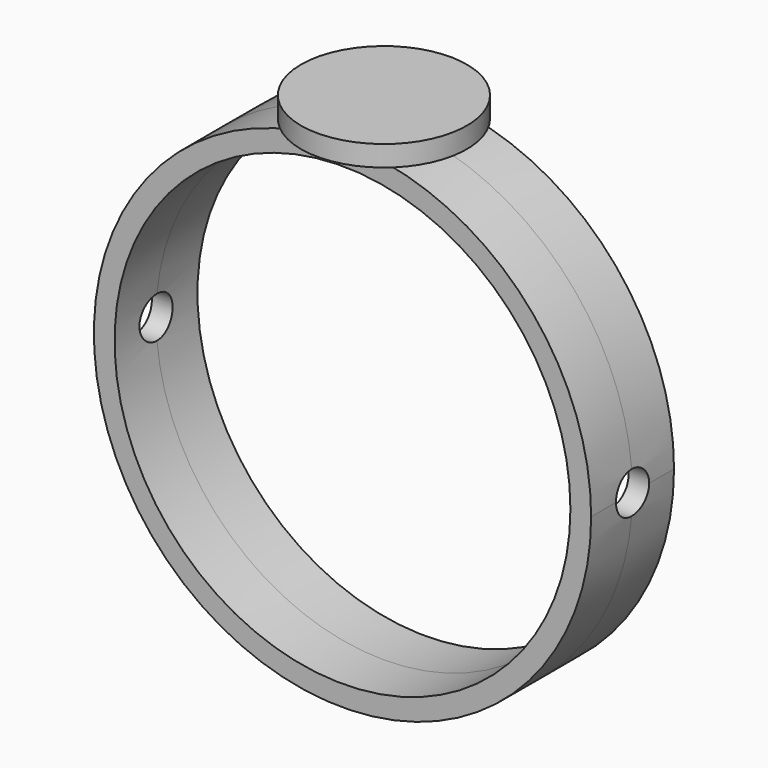
from build123d import *

# Parameters (mm, degrees)
F1_R     = 11
F2_DEPTH = 2.5
F1_W     = 4
F1_H     = 1
F4_R     = 1
F5_DEPTH = 30


with BuildPart() as f2:
    # F1 (on Front) → F2 (new body, symmetric)
    with BuildSketch(Plane.XZ):
        with BuildLine():
            ThreePointArc((0, 12), (-8.4852813742, -8.4852813742), (12, 0))
            ThreePointArc((12, 0), (8.4852813742, 8.4852813742), (0, 12))
        make_face()
        Circle(F1_R, mode=Mode.SUBTRACT)
    extrude(amount=F2_DEPTH, both=True)

    # F4 (on Right) → F5 (cut, symmetric)
    with BuildSketch(Plane.YZ):
        Circle(F4_R)
    extrude(amount=F5_DEPTH, both=True, mode=Mode.SUBTRACT)


with BuildPart() as f3:
    # F1 (on Front) → F3 (revolve)
    with BuildSketch(Plane.XZ):
        with Locations((-2, 12.5)):
            Rectangle(F1_W, F1_H)
    revolve(axis=Axis((0, 0, 12.5), (0, 0, 1)))


solid = Compound([f2.part, f3.part])
